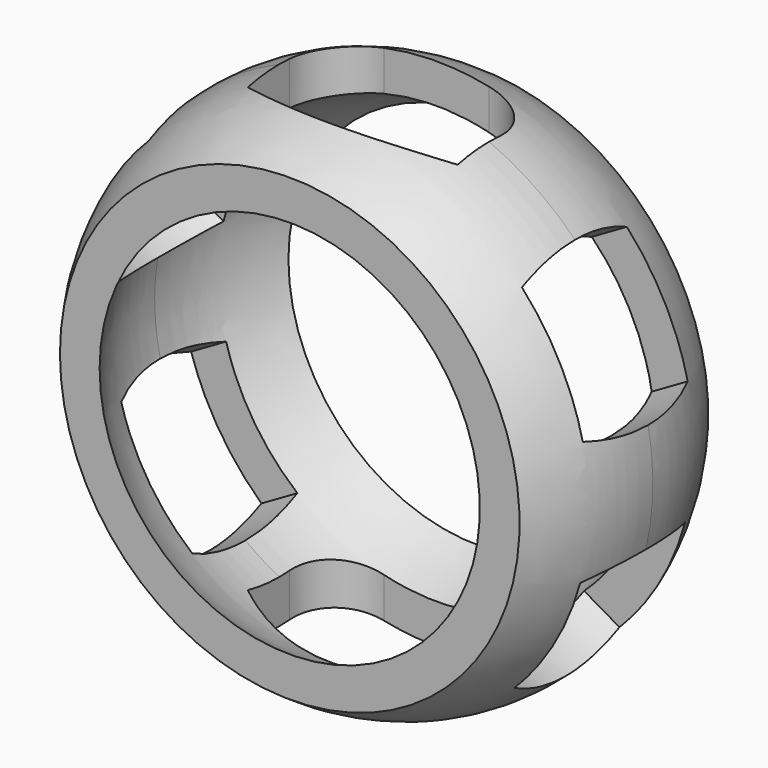
from build123d import *

# Parameters (mm, degrees)
F10_DEPTH = 228.6
F12_DEPTH = 228.6
F14_DEPTH = 228.6
F15_DEPTH = 228.6
F16_R     = 6.35
F17_DEPTH = 228.6


with BuildPart() as f1:
    # F0 (on Top) → F1 (revolve)
    with BuildSketch(Plane.XY):
        with BuildLine():
            ThreePointArc((-23.01875, -28.575), (-26.5592710348, -21.8176736783), (-27.78125, -14.2875))
            Line((-27.78125, -14.2875), (-32.53105, -14.2875))
            ThreePointArc((-32.53105, -14.2875), (-31.3241470584, -21.8092131032), (-27.82316, -28.575))
            Line((-27.82316, -28.575), (-23.01875, -28.575))
        make_face()
        with BuildLine():
            ThreePointArc((-27.78125, -14.2875), (-26.5592710348, -6.7573263217), (-23.01875, 0))
            Line((-23.01875, 0), (-27.81935, 0))
            ThreePointArc((-27.81935, 0), (-31.3223378245, -6.7654494374), (-32.53105, -14.2875))
            Line((-32.53105, -14.2875), (-27.78125, -14.2875))
        make_face()
    revolve(axis=Axis((0, -14.2875, 0), (0, -1, 0)))

    # F9 (on face) → F10 (cut)
    with BuildSketch(Plane(origin=(43.9940905122, 0, 25.4), x_dir=(0, -1, 0), z_dir=(-0.8660254038, 0, -0.5))):
        Polygon((6.35, 6.6849941881), (6.35, -1.2525058119), (6.35, -9.1900058119), (22.225, -9.1900058119), (22.225, -1.2525058119), (22.225, 6.6849941881), align=None)
        with BuildLine():
            Line((22.225, -9.1900058119), (6.35, -9.1900058119))
            ThreePointArc((6.35, -9.1900058119), (14.2875, -10.7726529787), (22.225, -9.1900058119))
        make_face()
        with BuildLine():
            ThreePointArc((22.225, 6.6849941881), (14.2875, 8.2676413549), (6.35, 6.6849941881))
            Line((6.35, 6.6849941881), (22.225, 6.6849941881))
        make_face()
    extrude(amount=F10_DEPTH, mode=Mode.SUBTRACT)

    # F11 (on face) → F12 (cut)
    with BuildSketch(Plane(origin=(43.9940905122, 0, -25.4), x_dir=(0, 1, 0), z_dir=(0.8660254038, 0, -0.5))):
        Polygon((-6.35, -7.9375), (-6.35, 0), (-6.35, 7.9375), (-22.225, 7.9375), (-22.225, 0), (-22.225, -7.9375), align=None)
    extrude(amount=-F12_DEPTH, mode=Mode.SUBTRACT)

    # F13 (on offset) → F14 (cut)
    with BuildSketch(Plane.XY.offset(-76.2)):
        Polygon((12.7, -6.35), (0, -6.35), (-12.7, -6.35), (-12.7, -19.05), (12.7, -19.05), align=None)
    extrude(amount=F14_DEPTH, mode=Mode.SUBTRACT)

    # F13 (on offset) → F15 (cut)
    with BuildSketch(Plane.XY.offset(-76.2)):
        Polygon((12.7, -6.35), (0, -6.35), (-12.7, -6.35), (-12.7, -19.05), (12.7, -19.05), align=None)
        with BuildLine():
            ThreePointArc((-12.7, -19.05), (0, -22.4529547439), (12.7, -19.05))
            Line((12.7, -19.05), (-12.7, -19.05))
        make_face()
    extrude(amount=F15_DEPTH, mode=Mode.SUBTRACT)

    # F16
    f16_edges = [f1.edges().sort_by_distance(p)[0] for p in [
        (-12.7, -6.35, -25.822114),
        (-12.7, -6.35, 25.822114),
        (12.7, -6.35, -25.822114),
        (12.7, -6.35, 25.822114),
    ]]
    fillet(f16_edges, radius=F16_R)

    # F11 (on face) → F17 (cut)
    with BuildSketch(Plane(origin=(43.9940905122, 0, -25.4), x_dir=(0, 1, 0), z_dir=(0.8660254038, 0, -0.5))):
        Polygon((-6.35, -7.9375), (-6.35, 0), (-6.35, 7.9375), (-22.225, 7.9375), (-22.225, 0), (-22.225, -7.9375), align=None)
        with BuildLine():
            ThreePointArc((-22.225, -7.9375), (-14.2875, -9.7702582843), (-6.35, -7.9375))
            Line((-6.35, -7.9375), (-22.225, -7.9375))
        make_face()
        with BuildLine():
            Line((-22.225, 7.9375), (-6.35, 7.9375))
            ThreePointArc((-6.35, 7.9375), (-14.2875, 9.5039686704), (-22.225, 7.9375))
        make_face()
    extrude(amount=-F17_DEPTH, mode=Mode.SUBTRACT)


solid = f1.part
